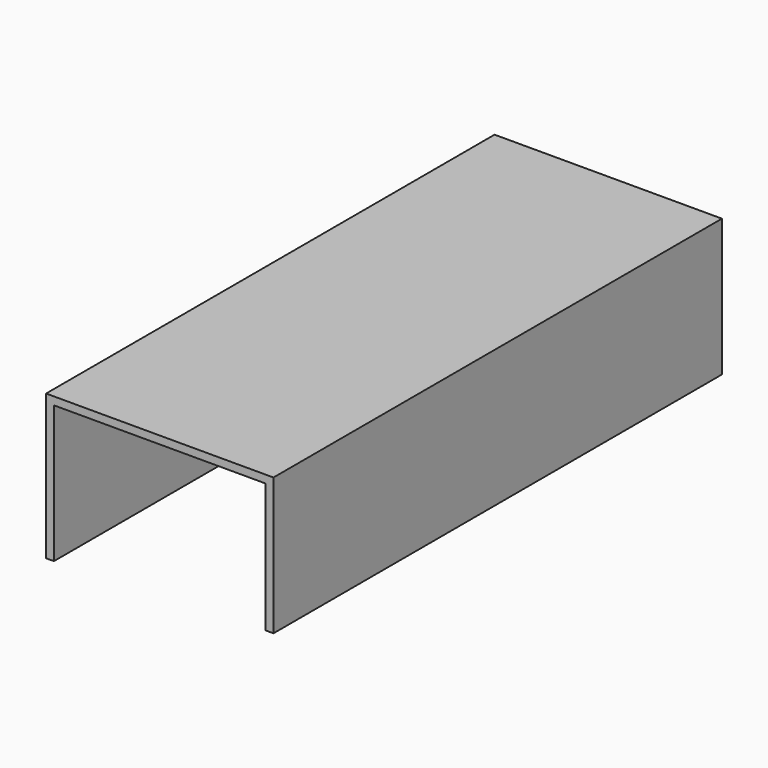
from build123d import *

# Parameters (mm, degrees)
F1_DEPTH = 143


# Not quite as in the source:
# - the program builds the solid bodies; features that only make, move or delete a surface that nothing else refers to are left out


with BuildPart() as f1:
    # F0 (on Front) → F1 (new body)
    with BuildSketch(Plane.XZ):
        Polygon((0, 0), (2, 0), (2, 35), (56, 35), (56, 2), (58, 2), (58, 37), (0, 37), align=None)
    extrude(amount=F1_DEPTH)


solid = f1.part
